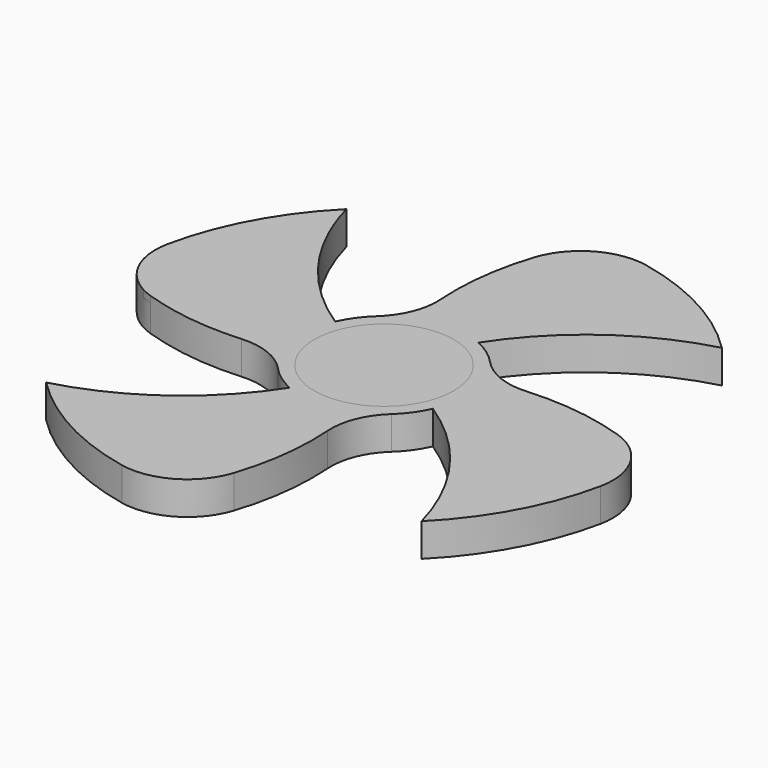
from build123d import *

# Parameters (mm, degrees)
F0_R     = 10.5
F1_DEPTH = 5
F2_R     = 10
F4_DEPTH = 1
F5_DEPTH = 1
F6_DEPTH = 5
F7_R     = 10


with BuildPart() as f1:
    # F0 (on Top) → F1 (new body)
    with BuildSketch(Plane.XY):
        with BuildLine():
            ThreePointArc((-11.6689185103, -4.481778754), (-12.4957774549, 0.3248781274), (-11.4202675565, 5.082075259))
            ThreePointArc((-11.4202675565, 5.082075259), (-22.0035263766, 15.1195796357), (-28.2842712475, 28.2842712475))
            ThreePointArc((-28.2842712475, 28.2842712475), (-36.9551813005, 15.3073372946), (-40, 0))
            ThreePointArc((-40, 0), (-26.25, -4.8676854218), (-11.6689185103, -4.481778754))
        make_face()
        with BuildLine():
            ThreePointArc((5.082075259, 11.4202675565), (15.1195796357, 22.0035263766), (28.2842712475, 28.2842712475))
            ThreePointArc((28.2842712475, 28.2842712475), (15.3073372946, 36.9551813005), (0, 40))
            ThreePointArc((0, 40), (-4.8676854218, 26.25), (-4.481778754, 11.6689185103))
            ThreePointArc((-4.481778754, 11.6689185103), (0.3248781274, 12.4957774549), (5.082075259, 11.4202675565))
        make_face()
        with BuildLine():
            ThreePointArc((11.6689185103, 4.481778754), (9.0655725015, 8.6061254476), (5.082075259, 11.4202675565))
            ThreePointArc((5.082075259, 11.4202675565), (0.3248781274, 12.4957774549), (-4.481778754, 11.6689185103))
            ThreePointArc((-4.481778754, 11.6689185103), (-8.6061254476, 9.0655725015), (-11.4202675565, 5.082075259))
            ThreePointArc((-11.4202675565, 5.082075259), (-12.4957774549, 0.3248781274), (-11.6689185103, -4.481778754))
            ThreePointArc((-11.6689185103, -4.481778754), (-9.0655725015, -8.6061254476), (-5.082075259, -11.4202675565))
            ThreePointArc((-5.082075259, -11.4202675565), (-0.3248781274, -12.4957774549), (4.481778754, -11.6689185103))
            ThreePointArc((4.481778754, -11.6689185103), (8.6061254476, -9.0655725015), (11.4202675565, -5.082075259))
            ThreePointArc((11.4202675565, -5.082075259), (12.2270876429, -2.597754371), (12.5, 0))
            ThreePointArc((12.5, 0), (12.2904735747, 2.2790917732), (11.6689185103, 4.481778754))
        make_face()
        Circle(F0_R, mode=Mode.SUBTRACT)
        with BuildLine():
            ThreePointArc((40, 0), (26.25, 4.8676854218), (11.6689185103, 4.481778754))
            ThreePointArc((11.6689185103, 4.481778754), (12.2904735747, 2.2790917732), (12.5, 0))
            ThreePointArc((12.5, 0), (12.2270876429, -2.597754371), (11.4202675565, -5.082075259))
            ThreePointArc((11.4202675565, -5.082075259), (22.0035263766, -15.1195796357), (28.2842712475, -28.2842712475))
            ThreePointArc((28.2842712475, -28.2842712475), (36.9551813005, -15.3073372946), (40, 0))
        make_face()
        with BuildLine():
            ThreePointArc((4.481778754, -11.6689185103), (-0.3248781274, -12.4957774549), (-5.082075259, -11.4202675565))
            ThreePointArc((-5.082075259, -11.4202675565), (-15.1195796357, -22.0035263766), (-28.2842712475, -28.2842712475))
            ThreePointArc((-28.2842712475, -28.2842712475), (-15.3073372946, -36.9551813005), (0, -40))
            ThreePointArc((0, -40), (4.8676854218, -26.25), (4.481778754, -11.6689185103))
        make_face()
    extrude(amount=F1_DEPTH)

    # F2
    f2_edges = [f1.edges().sort_by_distance(p)[0] for p in [
        (-40, 0, 2.5),
        (0, -40, 2.5),
        (40, 0, 2.5),
        (0, 40, 2.5),
    ]]
    fillet(f2_edges, radius=F2_R)

    # F3 (on face) → F4 (cut)
    with BuildSketch(Plane.XY.offset(5)):
        with BuildLine():
            ThreePointArc((-25.3116756684, -5.0047415232), (-25.3001707478, 5.0625806649), (-21.4369441775, 14.3591708391))
            ThreePointArc((-21.4369441775, 14.3591708391), (-23.9812309448, 18.1144371651), (-26.0839950043, 22.1336166391))
            ThreePointArc((-26.0839950043, 22.1336166391), (-32.548865417, 10.5282069215), (-34.1052807152, -2.6648842851))
            add(Edge.make_bspline(
                [(-34.1052807152, -2.6648842851), (-33.8455808028, -2.8046985599), (-33.5812223291, -2.9351651438), (-33.3126639182, -3.0560868057), (-33.040376273, -3.1672997314), (-32.7648420347, -3.2686740675), (-32.4865556414, -3.3601144662)],
                knots=[0.8783374065, 0.8783374065, 0.8783374065, 0.8783374065, 0.8783374065, 0.8783374065, 0.8783374065, 1, 1, 1, 1, 1, 1, 1], degree=6))
            ThreePointArc((-32.4865556414, -3.3601144662), (-28.9370274128, -4.347822521), (-25.3116756684, -5.0047415232))
        make_face()
    extrude(amount=-F4_DEPTH, mode=Mode.SUBTRACT)

    # F5 (add, through all): faces of the model
    f5_faces = [f1.faces().sort_by_distance(p)[0] for p in [
        (-28.4327754327, 7.5387813356, 4),
        (-28.4327754327, 7.5387813356, 4),
        (-28.4327754327, 7.5387813356, 4),
        (-28.4327754327, 7.5387813356, 4),
    ]]
    extrude(f5_faces, amount=F5_DEPTH)

    # F7
    f7_edges = [f1.edges().sort_by_distance(p)[0] for p in [
        (-11.668919, -4.481779, 2.5),
        (4.481779, -11.668919, 2.5),
        (11.668919, 4.481779, 2.5),
        (-4.481779, 11.668919, 2.5),
    ]]
    fillet(f7_edges, radius=F7_R)


with BuildPart() as f6:
    # F0 (on Top) → F6 (new body, through all)
    with BuildSketch(Plane.XY):
        Circle(F0_R)
    extrude(amount=F6_DEPTH)


solid = Compound([f1.part, f6.part])
